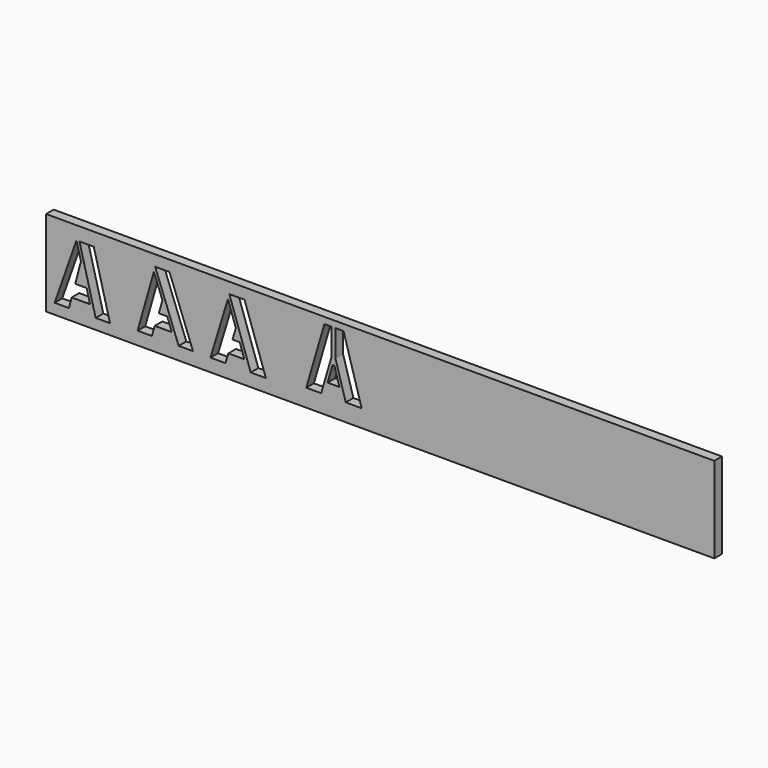
from build123d import *

# Parameters (mm, degrees)
F0_W     = 1778
F0_H     = 228.6
F1_DEPTH = 25.4
F3_DEPTH = 25.4
F5_DEPTH = 25.4
F7_DEPTH = 25.4
F9_DEPTH = 25.4


# Not quite as in the source:
# - a feature names something its author has since deleted; it is built from what else it names


with BuildPart() as f1:
    # F0 (on Front) → F1 (new body)
    with BuildSketch(Plane.XZ):
        with Locations((20.8893120289, -484.507374977)):
            Rectangle(F0_W, F0_H)
    extrude(amount=F1_DEPTH)

    # F2 (on face) → F3 (cut)
    with BuildSketch(Plane.XZ.offset(25.4)):
        Polygon((-787.2068197411, -405.6409977913), (-845.3705171574, -570.7409977913), (-807.2705171574, -570.7409977913), (-800.1682969996, -543.6377111227), (-751.1093717848, -543.6606517417), (-760.2752358596, -508.6147008675), (-790.3561904598, -508.6006346051), (-775.3030676873, -451.1553438794), align=None)
        Polygon((-779.3305171574, -405.6409977913), (-736.1505171574, -570.7409977913), (-698.0505171574, -570.7409977913), (-741.2305171574, -405.6409977913), align=None)
    extrude(amount=-F3_DEPTH, mode=Mode.SUBTRACT)

    # F4 (on face) → F5 (cut)
    with BuildSketch(Plane.XZ.offset(25.4)):
        Polygon((-577.868904515, -399.2722157273), (-515.3390834819, -564.3722157273), (-477.2390834819, -564.3722157273), (-539.768904515, -399.2722157273), align=None)
        Polygon((-581.2202315634, -411.9376221896), (-624.5590834819, -564.3722157273), (-586.4590834819, -564.3722157273), (-579.0069102806, -538.1608847247), (-533.414550058, -538.1608847247), (-545.856203928, -505.3106858916), (-568.1572882119, -505.3106858916), (-558.5947445746, -471.6766049683), align=None)
    extrude(amount=-F5_DEPTH, mode=Mode.SUBTRACT)

    # F6 (on face) → F7 (cut)
    with BuildSketch(Plane.XZ.offset(25.4)):
        Polygon((-384.2945505557, -411.7044204948), (-430.6923954532, -564.3722157273), (-390.8717237614, -564.3722157273), (-383.1523140548, -538.9722157273), (-372.2040461495, -502.9479579969), (-363.142928275, -473.133192003), align=None)
        Polygon((-372.2040461495, -502.9479579969), (-383.1523140548, -538.9722157273), (-340.4727343746, -538.9722157273), (-352.8768810595, -502.9479579969), align=None)
        Polygon((-340.2208844074, -399.2722157273), (-380.5162323606, -399.2722157273), (-323.6677434064, -564.3722157273), (-283.3723954532, -564.3722157273), align=None)
    extrude(amount=-F7_DEPTH, mode=Mode.SUBTRACT)

    # F8 (on face) → F9 (cut)
    with BuildSketch(Plane.XZ.offset(25.4)):
        Polygon((-108.2167720242, -386.9905862627), (-127.4883288311, -386.9506543679), (-175.7540198106, -551.9509992015), (-136.0814640163, -552.0332032675), (-108.3624021802, -457.2732471037), align=None)
        Polygon((-105.9366706351, -476.1219167204), (-119.2716706351, -521.7087415168), (-87.5217387934, -521.7745294006), (-100.8566706351, -476.1219167204), align=None)
        Polygon((-28.4340198106, -552.2562556378), (-76.6883288311, -387.055915208), (-98.2782824835, -387.011179447), (-98.4238699691, -457.2732471037), (-70.7053259606, -552.1686667953), align=None)
    extrude(amount=-F9_DEPTH, mode=Mode.SUBTRACT)


solid = f1.part
